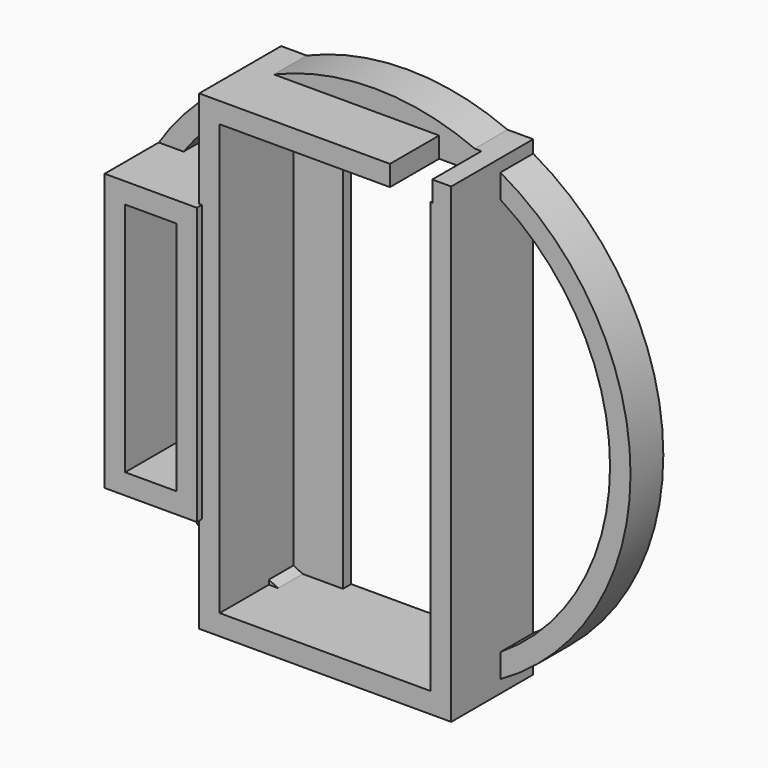
from build123d import *

# Parameters (mm, degrees)
F1_DEPTH      = 5.08
F2_W          = 31.242
F2_H          = 58.42
F2_W_2        = 26.162
F2_H_2        = 53.34
F3_DEPTH      = 12.7
F6_W          = 31.242
F6_H          = 58.42
F7_DEPTH      = 1.27
F8_W          = 11.43
F8_H          = 34.29
F9_DEPTH      = 8.382
F10_T         = 2.54
F10_T3_DEPTH  = 10.16
F10_T5_DEPTH  = 8.153909223
F10_T7_DEPTH  = 5.4081357261
F10_T9_DEPTH  = 39.37
F10_T11_DEPTH = 8.0392489691
F10_T13_DEPTH = 17.78
F10_T15_DEPTH = 8.0392489691
F10_T17_DEPTH = 29.9668157867
F10_T19_DEPTH = 8.89
F10_T21_DEPTH = 28.9073120599
F10_T23_DEPTH = 6.24734397
F10_T25_DEPTH = 12.7
F10_T27_DEPTH = 6.24734397
F10_T29_DEPTH = 57.3145303032
F10_T31_DEPTH = 5.6327348484
F10_T33_DEPTH = 5.6327348484
F10_T36_ANGLE = 2.5336786408
F10_T38_ANGLE = 2.5336786408
F10_T40_ANGLE = 2.5336786408
F10_T42_ANGLE = 2.5336786408
F11_W         = 13.877093792
F11_H         = 53.34
F12_DEPTH     = 25.4
F14_DEPTH     = 7.62
F16_DEPTH     = 1.778


# Not quite as in the source:
# - a feature of the source that left no trace in its solid (it failed there, or was rolled back) is left out
# - a shell that OpenCascade refuses in one call is made with other operations: the cavity is built on its own and cut out


with BuildPart() as f1:
    # F0 (on Front) → F1 (new body)
    with BuildSketch(Plane.XZ):
        with BuildLine():
            Line((-26.7228642739, 17.145), (-26.7228642739, -17.145))
            ThreePointArc((-26.7228642739, -17.145), (31.75, 0), (-26.7228642739, 17.145))
        make_face()
        with BuildLine():
            ThreePointArc((-24.1828642739, 16.3833200393), (29.21, 0), (-24.1828642739, -16.3833200393))
            Line((-24.1828642739, -16.3833200393), (-24.1828642739, 16.3833200393))
        make_face(mode=Mode.SUBTRACT)
    extrude(amount=F1_DEPTH)

    # F2 (on Front) → F3 (join)
    with BuildSketch(Plane.XZ):
        Rectangle(F2_W, F2_H)
        Rectangle(F2_W_2, F2_H_2, mode=Mode.SUBTRACT)
    extrude(amount=F3_DEPTH)

    # F6 (on Front) → F7 (join)
    with BuildSketch(Plane.XZ):
        Rectangle(F6_W, F6_H)
    extrude(amount=F7_DEPTH)

    # F8 (on face) → F9 (join, symmetric)
    with BuildSketch(Plane.XZ.offset(5.08)):
        with Locations((-21.0078642739, 0)):
            Rectangle(F8_W, F8_H)
    extrude(amount=F9_DEPTH, both=True)

    # F10: shell of thickness 2.54, made by hand


with BuildPart() as f10_core1:
    # F10_t2: copy of F1
    add(f1.part)

    # the walls: a layer under each face that stays
    f10_faces = [f10_core1.faces().sort_by_distance(p)[0] for p in [
        (-26.7228642739, -5.08, 0),
        (-21.8127096171, -2.54, 23.0709384109),
        (-21.8127096171, -2.54, -23.0709384109),
        (2.5135678631, 0, 0),
        (-15.621, -6.35, 23.1775),
        (-21.1719321369, -5.08, 22.3931987794),
        (-21.1719321369, -5.08, -22.3931987794),
        (-15.621, -6.35, -23.1775),
        (-21.0078642739, -5.08, 17.145),
        (-21.0078642739, -5.08, -17.145),
        (-21.0078642739, 3.302, 0),
        (0, -6.35, 29.21),
        (0, -2.54, 31.75),
        (15.621, -6.35, 0),
        (31.75, -2.54, 0),
        (0, -6.35, -29.21),
        (0, -2.54, -31.75),
        (-19.9933612642, -2.54, -21.2952953809),
        (-15.2928642739, 1.651, 0),
        (-19.9933612642, -2.54, 21.2952953809),
        (29.21, -2.54, 0),
        (-13.3894285714, -12.7, -25.0371428571),
        (-15.2928642739, -13.081, 0),
        (0, -5.08, 30.48),
        (23.6855, -5.08, -18.4275983725),
        (0, -5.08, -30.48),
        (0, -6.985, 26.67),
        (-13.081, -6.985, 0),
        (13.081, -6.985, 0),
        (0, -6.985, -26.67),
        (-12.5003834528, -3.175, 26.4000854834),
        (0, -1.27, 0),
        (12.5003834528, -3.175, 26.4000854834),
        (12.497328015, -5.08, 26.5778775253),
        (-12.8864426717, -5.08, 26.3936325758),
        (-12.5003834528, -3.175, -26.4000854834),
        (-12.8864426717, -5.08, -26.5778775253),
        (12.5003834528, -3.175, -26.4000854834),
        (12.497328015, -5.08, -26.5778775253),
    ]]
    thicken(f10_faces, amount=-F10_T, mode=Mode.SUBTRACT)

    # F10_s4 → F10_t3 (cut)
    with BuildSketch(Plane.XZ.offset(-2.54)):
        Polygon((-15.6588968, 27.6635106768), (-14.37132, 25.430085754), (-13.081, 26.1592850891), (-13.081, 27.6413975587), align=None)
        Polygon((-15.6588968, -27.6635106768), (-14.37132, -25.430085754), (-13.081, -26.1592850891), (-13.081, -27.6413975587), align=None)
        Polygon((-15.6328165217, 24.6606858517), (-13.081, 24.6821485896), (-13.081, 29.2956343073), (-16.9793478261, 26.82842238), align=None)
        Polygon((-15.6328165217, -24.6606858517), (-13.081, -24.6821485896), (-13.081, -29.2956343073), (-16.9793478261, -26.82842238), align=None)
        Polygon((-23.6283907422, 17.1554913043), (-23.6489550509, 14.605), (-28.62768243, 14.605), (-25.7053859249, 18.6358695652), align=None)
        Polygon((-23.6283907422, -17.1554913043), (-23.6489550509, -14.605), (-28.62768243, -14.605), (-25.7053859249, -18.6358695652), align=None)
        Polygon((12.4533626197, 29.258768), (12.4434078933, 26.67), (11.9249325645, 26.67), (11.4479352619, 26.8732), align=None)
        Polygon((-12.4533626197, 29.258768), (-12.4434078933, 26.67), (-11.9249325644, 26.67), (-11.4479352619, 26.8732), align=None)
        Polygon((15.6588968, 27.6635106768), (13.081, 27.6413975587), (13.081, 26.1592850891), (14.37132, 25.430085754), align=None)
        Polygon((15.6328165217, 24.6606858517), (13.081, 24.6821485896), (13.081, 29.2956343073), (16.9793478261, 26.82842238), align=None)
        Polygon((15.6328165217, -24.6606858517), (13.081, -24.6821485896), (13.081, -29.2956343073), (16.9793478261, -26.82842238), align=None)
        Polygon((15.6588968, -27.6635106768), (13.081, -27.6413975587), (13.081, -26.1592850891), (14.37132, -25.430085754), align=None)
        Polygon((-12.4533626197, -29.258768), (-12.4434078933, -26.67), (-11.9249325645, -26.67), (-11.4479352619, -26.8732), align=None)
        Polygon((12.4533626197, -29.258768), (12.4434078933, -26.67), (11.9249325644, -26.67), (11.4479352619, -26.8732), align=None)
    extrude(amount=F10_T3_DEPTH, mode=Mode.SUBTRACT)

    # F10_s6 → F10_t5 (cut)
    with BuildSketch(Plane.YZ.offset(-29.2628642739)):
        Polygon((0.0254, 17.1704), (-2.54, 17.145), (-2.54, 14.605), (0, 14.605), align=None)
        Polygon((0.0254, -17.1704), (-2.54, -17.145), (-2.54, -14.605), (0, -14.605), align=None)
        Polygon((-5.1054, 17.1704), (-2.54, 17.145), (-2.54, 14.605), (-5.08, 14.605), align=None)
        Polygon((-5.1054, -17.1704), (-2.54, -17.145), (-2.54, -14.605), (-5.08, -14.605), align=None)
    extrude(amount=F10_T5_DEPTH, mode=Mode.SUBTRACT)

    # F10_s8 → F10_t7 (cut)
    with BuildSketch(Plane.YZ.offset(-18.161)):
        Polygon((0.0254, -17.1704), (-2.54, -17.145), (-2.54, -14.605), (0, -14.605), align=None)
        Polygon((0.0254, 17.1704), (-2.54, 17.145), (-2.54, 14.605), (0, 14.605), align=None)
        Polygon((-12.7254, 17.1704), (-12.7, 14.605), (-10.16, 14.605), (-10.16, 17.145), align=None)
        Polygon((-12.7254, -17.1704), (-12.7, -14.605), (-10.16, -14.605), (-10.16, -17.145), align=None)
    extrude(amount=F10_T7_DEPTH, mode=Mode.SUBTRACT)

    # F10_s10 → F10_t9 (cut)
    with BuildSketch(Plane.XY.offset(-19.685)):
        Polygon((-15.2674642739, 0.0254), (-15.2928642739, -2.54), (-17.8328642739, -2.54), (-17.8328642739, 0), align=None)
        Polygon((-15.2674642739, -12.7254), (-15.2928642739, -10.16), (-17.8328642739, -10.16), (-17.8328642739, -12.7), align=None)
    extrude(amount=F10_T9_DEPTH, mode=Mode.SUBTRACT)

    # F10_s12 → F10_t11 (cut)
    with BuildSketch(Plane.XY.offset(22.1421485896)):
        Polygon((-15.6464, -5.1054), (-13.081, -5.08), (-13.081, -2.54), (-15.621, -2.54), align=None)
        Polygon((15.6464, -5.1054), (13.081, -5.08), (13.081, -2.54), (15.621, -2.54), align=None)
    extrude(amount=F10_T11_DEPTH, mode=Mode.SUBTRACT)

    # F10_s14 → F10_t13 (cut)
    with BuildSketch(Plane.XZ.offset(-2.54)):
        Polygon((-15.6464, 17.1704), (-13.081, 17.145), (-13.081, 14.605), (-15.621, 14.605), align=None)
        Polygon((-15.6464, -17.1704), (-13.081, -17.145), (-13.081, -14.605), (-15.621, -14.605), align=None)
    extrude(amount=F10_T13_DEPTH, mode=Mode.SUBTRACT)

    # F10_s16 → F10_t15 (cut)
    with BuildSketch(Plane.XY.offset(-30.1813975587)):
        Polygon((-15.6464, -5.1054), (-15.621, -2.54), (-13.081, -2.54), (-13.081, -5.08), align=None)
        Polygon((15.6464, -5.1054), (13.081, -5.08), (13.081, -2.54), (15.621, -2.54), align=None)
    extrude(amount=F10_T15_DEPTH, mode=Mode.SUBTRACT)

    # F10_s18 → F10_t17 (cut)
    with BuildSketch(Plane.YZ.offset(-14.9834078933)):
        Polygon((-5.1054, 29.2354), (-5.08, 26.67), (-2.54, 26.67), (-2.54, 29.21), align=None)
        Polygon((-5.1054, -29.2354), (-5.08, -26.67), (-2.54, -26.67), (-2.54, -29.21), align=None)
    extrude(amount=F10_T17_DEPTH, mode=Mode.SUBTRACT)

    # F10_s20 → F10_t19 (cut)
    with BuildSketch(Plane.XZ.offset(-1.27)):
        Polygon((-11.9032963291, 26.6214086957), (-11.91365603, 29.21), (-12.4551858495, 29.21), (-12.9496261195, 28.9891304348), align=None)
        Polygon((11.9032963291, 26.6214086957), (11.91365603, 29.21), (12.4551858495, 29.21), (12.9496261195, 28.9891304348), align=None)
        Polygon((-13.0442252174, -26.0945544863), (-15.621, -26.1172651516), (-15.621, -27.6858696652), (-14.2184782609, -28.3883316865), align=None)
        Polygon((-13.0442252174, 26.0945544863), (-15.621, 26.1172651516), (-15.621, 27.6858696652), (-14.2184782609, 28.3883316865), align=None)
        Polygon((13.0442252174, 26.0945544863), (15.621, 26.1172651516), (15.621, 27.6858696652), (14.2184782609, 28.3883316865), align=None)
        Polygon((13.0442252174, -26.0945544863), (15.621, -26.1172651516), (15.621, -27.6858696652), (14.2184782609, -28.3883316865), align=None)
        Polygon((11.9032963291, -26.6214086957), (11.91365603, -29.21), (12.4551858495, -29.21), (12.9496261195, -28.9891304348), align=None)
        Polygon((-11.9032963291, -26.6214086957), (-11.91365603, -29.21), (-12.4551858495, -29.21), (-12.9496261195, -28.9891304348), align=None)
    extrude(amount=F10_T19_DEPTH, mode=Mode.SUBTRACT)

    # F10_s22 → F10_t21 (cut)
    with BuildSketch(Plane.YZ.offset(-14.45365603)):
        Polygon((-1.2954, 26.6446), (-1.27, 29.21), (1.27, 29.21), (1.27, 26.67), align=None)
        Polygon((-1.2954, -26.6446), (-1.27, -29.21), (1.27, -29.21), (1.27, -26.67), align=None)
    extrude(amount=F10_T21_DEPTH, mode=Mode.SUBTRACT)

    # F10_s24 → F10_t23 (cut)
    with BuildSketch(Plane.YZ.offset(9.37365603)):
        Polygon((-5.1054, 26.6446), (-5.08, 29.21), (-2.54, 29.21), (-2.54, 26.67), align=None)
        Polygon((-5.1054, -26.6446), (-5.08, -29.21), (-2.54, -29.21), (-2.54, -26.67), align=None)
    extrude(amount=F10_T23_DEPTH, mode=Mode.SUBTRACT)

    # F10_s26 → F10_t25 (cut)
    with BuildSketch(Plane.XZ.offset(2.54)):
        Polygon((13.0556, 26.6446), (13.081, 29.21), (15.621, 29.21), (15.621, 26.67), align=None)
        Polygon((-13.0556, 26.6446), (-13.081, 29.21), (-15.621, 29.21), (-15.621, 26.67), align=None)
        Polygon((-13.0556, -26.6446), (-15.621, -26.67), (-15.621, -29.21), (-13.081, -29.21), align=None)
        Polygon((13.0556, -26.6446), (15.621, -26.67), (15.621, -29.21), (13.081, -29.21), align=None)
    extrude(amount=F10_T25_DEPTH, mode=Mode.SUBTRACT)

    # F10_s28 → F10_t27 (cut)
    with BuildSketch(Plane.YZ.offset(-15.621)):
        Polygon((-5.1054, 26.6446), (-5.08, 29.21), (-2.54, 29.21), (-2.54, 26.67), align=None)
        Polygon((-5.1054, -26.6446), (-5.08, -29.21), (-2.54, -29.21), (-2.54, -26.67), align=None)
    extrude(amount=F10_T27_DEPTH, mode=Mode.SUBTRACT)

    # F10_s30 → F10_t29 (cut)
    with BuildSketch(Plane.XY.offset(-28.6572651516)):
        Polygon((-13.0556, -1.2954), (-15.621, -1.27), (-15.621, 1.27), (-13.081, 1.27), align=None)
        Polygon((13.0556, -1.2954), (15.621, -1.27), (15.621, 1.27), (13.081, 1.27), align=None)
    extrude(amount=F10_T29_DEPTH, mode=Mode.SUBTRACT)

    # F10_s32 → F10_t31 (cut)
    with BuildSketch(Plane.XY.offset(23.5772651516)):
        Polygon((-13.0556, -5.1054), (-15.621, -5.08), (-15.621, -2.54), (-13.081, -2.54), align=None)
        Polygon((13.0556, -5.1054), (15.621, -5.08), (15.621, -2.54), (13.081, -2.54), align=None)
    extrude(amount=F10_T31_DEPTH, mode=Mode.SUBTRACT)

    # F10_s34 → F10_t33 (cut)
    with BuildSketch(Plane.XY.offset(-29.21)):
        Polygon((-13.0556, -5.1054), (-15.621, -5.08), (-15.621, -2.54), (-13.081, -2.54), align=None)
        Polygon((13.0556, -5.1054), (15.621, -5.08), (15.621, -2.54), (13.081, -2.54), align=None)
    extrude(amount=F10_T33_DEPTH, mode=Mode.SUBTRACT)

    # F10_s35 → F10_t36 (revolve, cut)
    with BuildSketch(Plane(origin=(0, 0, 0), x_dir=(0, 1, 0), z_dir=(-0.894120683, 0, -0.447826087))):
        Polygon((-1.2954, -29.1846), (-1.27, -31.75), (1.27, -31.75), (1.27, -29.21), align=None)
    revolve(axis=Axis((0, -1.27, 0), (0, 1, 0)), revolution_arc=F10_T36_ANGLE, mode=Mode.SUBTRACT)

    # F10_s37 → F10_t38 (revolve, cut)
    with BuildSketch(Plane(origin=(0, 0, 0), x_dir=(0, 1, 0), z_dir=(-0.9130434783, 0, 0.40786224))):
        Polygon((-1.2954, -29.1846), (1.27, -29.21), (1.27, -31.75), (-1.27, -31.75), align=None)
    revolve(axis=Axis((0, -1.27, 0), (0, 1, 0)), revolution_arc=F10_T38_ANGLE, mode=Mode.SUBTRACT)

    # F10_s39 → F10_t40 (revolve, cut)
    with BuildSketch(Plane(origin=(0, 0, 0), x_dir=(0, 1, 0), z_dir=(0.894120683, 0, 0.447826087))):
        Polygon((-1.2954, -29.1846), (1.27, -29.21), (1.27, -31.75), (-1.27, -31.75), align=None)
    revolve(axis=Axis((0, -1.27, 0), (0, 1, 0)), revolution_arc=F10_T40_ANGLE, mode=Mode.SUBTRACT)

    # F10_s41 → F10_t42 (revolve, cut)
    with BuildSketch(Plane(origin=(0, 0, 0), x_dir=(0, 1, 0), z_dir=(0.9130434783, 0, -0.40786224))):
        Polygon((-1.2954, -29.1846), (1.27, -29.21), (1.27, -31.75), (-1.27, -31.75), align=None)
    revolve(axis=Axis((0, -1.27, 0), (0, 1, 0)), revolution_arc=F10_T42_ANGLE, mode=Mode.SUBTRACT)


with BuildPart() as f1_1:
    add(f1.part)

    # what is left inside the walls is the cavity
    f10_cavity = [f10_core1.part.solids().sort_by_distance(p)[0] for p in [
        (-24.157464, -8.720667, 0),
    ]]
    add(f10_cavity, mode=Mode.SUBTRACT)

    # F11 (on face) → F12 (cut)
    with BuildSketch(Plane.XZ.offset(1.27)):
        Rectangle(F11_W, F11_H)
    extrude(amount=-F12_DEPTH, mode=Mode.SUBTRACT)

    # F13 (on face) → F14 (cut)
    with BuildSketch(Plane.XZ.offset(12.7)):
        Polygon((13.2733471692, 26.67), (13.2733471692, 29.21), (8.0283172429, 29.21), (8.0283172429, 26.67), (13.081, 26.67), align=None)
    extrude(amount=-F14_DEPTH, mode=Mode.SUBTRACT)

    # F15 (on face) → F16 (cut)
    with BuildSketch(Plane(origin=(-26.7228642739, 0, 0), x_dir=(0, -1, 0), z_dir=(-1, 0, 0))):
        with BuildLine():
            Line((8.7604723504, 0), (7.1624774839, 14.2667547511))
            ThreePointArc((7.1624774839, 14.2667547511), (6.4768419594, 15.5955348237), (5.08, 16.129))
            ThreePointArc((5.08, 16.129), (3.6831580406, 15.5955348237), (2.9975225161, 14.2667547511))
            Line((2.9975225161, 14.2667547511), (1.3995276496, 0))
            Line((1.3995276496, 0), (2.9975225161, -14.2667547511))
            ThreePointArc((2.9975225161, -14.2667547511), (3.6831580406, -15.5955348237), (5.08, -16.129))
            ThreePointArc((5.08, -16.129), (6.4768419594, -15.5955348237), (7.1624774839, -14.2667547511))
            Line((7.1624774839, -14.2667547511), (8.7604723504, 0))
        make_face()
    extrude(amount=-F16_DEPTH, mode=Mode.SUBTRACT)


solid = f1_1.part
